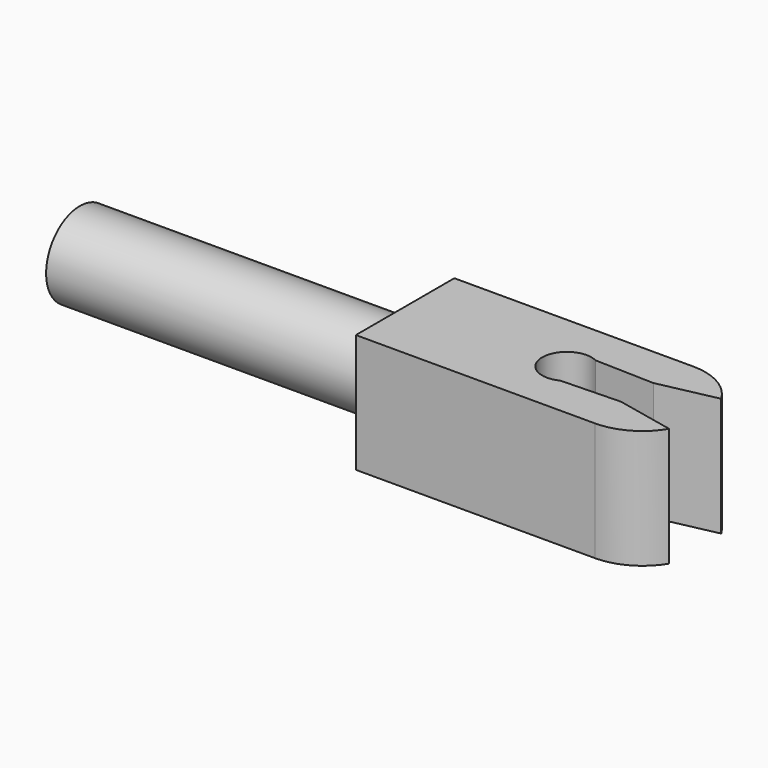
from build123d import *

# Parameters (mm, degrees)
F1_DEPTH      = 3.375
F1_DEPTH_BACK = 3.375
F2_R          = 2.4
F3_DEPTH      = 18.5
F4_T1_DEPTH   = 21.2682356522


# Not quite as in the source:
# - a fillet or chamfer that OpenCascade refuses, or shapes differently, is made with other operations: its cross-section is extruded or revolved along the edge and cut away or added


with BuildPart() as f1:
    # F0 (on Top) → F1 (new body, two sides)
    with BuildSketch(Plane.XY) as f1_sk:
        with BuildLine():
            Line((16.5, 3.5), (0, 3.5))
            Line((0, 3.5), (0, 2.35))
            Line((0, 2.35), (0, -2.35))
            Line((0, -2.35), (0, -3.5))
            Line((0, -3.5), (16.5, -3.5))
            Line((16.5, -3.5), (16.5, -1.85))
            Line((16.5, -1.85), (13.2, -1.15))
            Line((13.2, -1.15), (9.8304760106, -1.25))
            ThreePointArc((9.8304760106, -1.25), (7.8, 0), (9.8304760106, 1.25))
            Line((9.8304760106, 1.25), (13.2, 1.15))
            Line((13.2, 1.15), (16.5, 1.85))
            Line((16.5, 1.85), (16.5, 3.5))
        make_face()
    extrude(amount=F1_DEPTH)
    extrude(f1_sk.sketch, amount=-F1_DEPTH_BACK)

    # F2 (on face) → F3 (join)
    with BuildSketch(Plane(origin=(0, 0, 0), x_dir=(0, -1, 0), z_dir=(-1, 0, 0))):
        Circle(F2_R)
    extrude(amount=F3_DEPTH)

    # F4: fillet of radius 3.3798989873 on 2 edges, made by hand

    # F4_s2 → F4_t1 (cut)
    with BuildSketch(Plane.XY.offset(-10.6341178261)):
        with BuildLine():
            ThreePointArc((13.5963528696, -3.5), (15.2662081521, -3.0586891941), (16.5, -1.85))
            Line((16.5, -1.85), (16.5, -3.5))
            Line((16.5, -3.5), (13.5963528696, -3.5))
        make_face()
        with BuildLine():
            ThreePointArc((16.5, 1.85), (15.2662081521, 3.0586891941), (13.5963528696, 3.5))
            Line((13.5963528696, 3.5), (16.5, 3.5))
            Line((16.5, 3.5), (16.5, 1.85))
        make_face()
    extrude(amount=F4_T1_DEPTH, mode=Mode.SUBTRACT)


solid = f1.part
